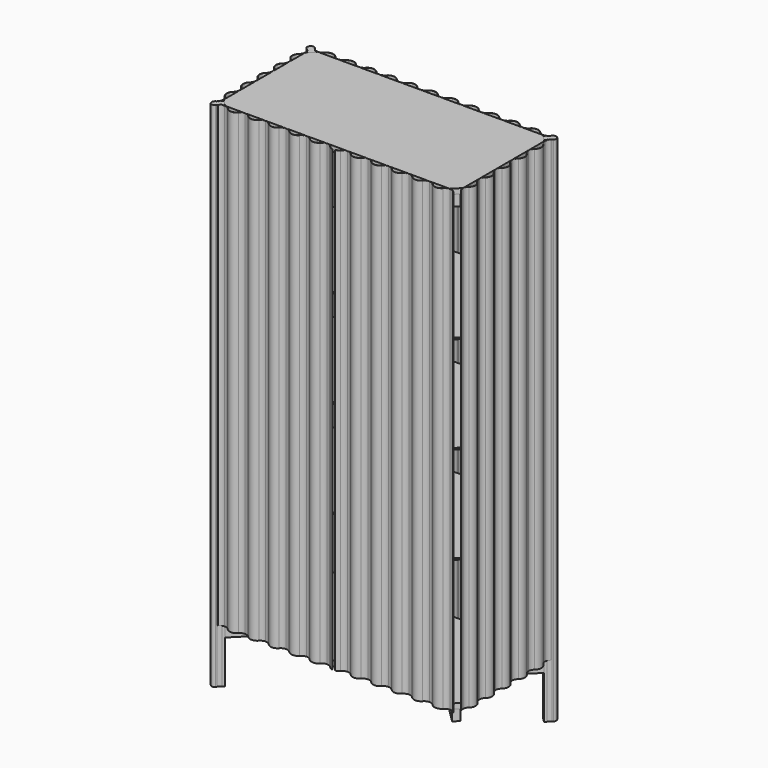
from build123d import *

# Parameters (mm, degrees)
F1_DEPTH       = 1700
F1_DEPTH_BACK  = 200
F2_DEPTH       = 1700
F4_DEPTH       = 19
F7_DEPTH       = 40
F8_DEPTH       = 40
F12_DEPTH      = 3
F12_DEPTH_BACK = 3
F15_R          = 2
F16_DEPTH      = 341.9145833847
F16_DEPTH_BACK = 642.3552756058


# Not quite as in the source:
# - a feature names something its author has since deleted; it is built from what else it names


with BuildPart() as f1:
    # F0 (on Top) → F1 (new body, two sides)
    with BuildSketch(Plane.XY) as f1_sk:
        with BuildLine():
            Line((-444.1128755262, -200.5565263401), (-451.3698203647, -207.8134711786))
            Line((-451.3698203647, -207.8134711786), (-454.0123704628, -210.4560212767))
            Line((-454.0123704628, -210.4560212767), (-455.0730306346, -209.3953611049))
            Line((-455.0730306346, -209.3953611049), (-458.3300735629, -212.6524040333))
            ThreePointArc((-458.3300735629, -212.6524040333), (-458.3300735629, -230.3300735629), (-440.6524040333, -230.3300735629))
            Line((-440.6524040333, -230.3300735629), (-437.3953611049, -227.0730306346))
            Line((-437.3953611049, -227.0730306346), (-438.4560212767, -226.0123704628))
            Line((-438.4560212767, -226.0123704628), (-435.8134706741, -223.3698198602))
            Line((-435.8134706741, -223.3698198602), (-428.5565263401, -216.1128755262))
            Line((-428.5565263401, -216.1128755262), (-427.4958661683, -217.1735356979))
            Line((-427.4958661683, -217.1735356979), (-421.2069675506, -210.8846370803))
            Line((-421.2069675506, -210.8846370803), (-438.8846370803, -193.2069675506))
            Line((-438.8846370803, -193.2069675506), (-445.1735356979, -199.4958661683))
            Line((-445.1735356979, -199.4958661683), (-444.1128755262, -200.5565263401))
        make_face()
    extrude(amount=F1_DEPTH)
    extrude(f1_sk.sketch, amount=-F1_DEPTH_BACK)


with BuildPart() as f1b:
    # F0 (on Top) → F1, piece 2 (new body, two sides)
    with BuildSketch(Plane.XY) as f1_2_sk:
        with BuildLine():
            Line((-428.5565263401, 216.1128755262), (-435.8134706741, 223.3698198602))
            Line((-435.8134706741, 223.3698198602), (-438.4560212767, 226.0123704628))
            Line((-438.4560212767, 226.0123704628), (-437.3953611049, 227.0730306346))
            Line((-437.3953611049, 227.0730306346), (-440.6524040333, 230.3300735629))
            ThreePointArc((-440.6524040333, 230.3300735629), (-458.3300735629, 230.3300735629), (-458.3300735629, 212.6524040333))
            Line((-458.3300735629, 212.6524040333), (-455.0730306346, 209.3953611049))
            Line((-455.0730306346, 209.3953611049), (-454.0123704628, 210.4560212767))
            Line((-454.0123704628, 210.4560212767), (-451.3698200275, 207.8134708414))
            Line((-451.3698200275, 207.8134708414), (-444.1128755262, 200.5565263401))
            Line((-444.1128755262, 200.5565263401), (-445.1735356979, 199.4958661683))
            Line((-445.1735356979, 199.4958661683), (-438.8846370803, 193.2069675506))
            Line((-438.8846370803, 193.2069675506), (-421.2069675506, 210.8846370803))
            Line((-421.2069675506, 210.8846370803), (-427.4958661683, 217.1735356979))
            Line((-427.4958661683, 217.1735356979), (-428.5565263401, 216.1128755262))
        make_face()
    extrude(amount=F1_DEPTH)
    extrude(f1_2_sk.sketch, amount=-F1_DEPTH_BACK)


with BuildPart() as f1c:
    # F0 (on Top) → F1, piece 3 (new body, two sides)
    with BuildSketch(Plane.XY) as f1_3_sk:
        with BuildLine():
            Line((438.4560212767, 226.0123704628), (435.8134711117, 223.3698202978))
            Line((435.8134711117, 223.3698202978), (428.5565263401, 216.1128755262))
            Line((428.5565263401, 216.1128755262), (427.4958661683, 217.1735356979))
            Line((427.4958661683, 217.1735356979), (421.2069675506, 210.8846370803))
            Line((421.2069675506, 210.8846370803), (438.8846370803, 193.2069675506))
            Line((438.8846370803, 193.2069675506), (445.1735356979, 199.4958661683))
            Line((445.1735356979, 199.4958661683), (444.1128755262, 200.5565263401))
            Line((444.1128755262, 200.5565263401), (451.3698203996, 207.8134712135))
            Line((451.3698203996, 207.8134712135), (454.0123704628, 210.4560212767))
            Line((454.0123704628, 210.4560212767), (455.0730306346, 209.3953611049))
            Line((455.0730306346, 209.3953611049), (458.3300735629, 212.6524040333))
            ThreePointArc((458.3300735629, 212.6524040333), (458.3300735629, 230.3300735629), (440.6524040333, 230.3300735629))
            Line((440.6524040333, 230.3300735629), (437.3953611049, 227.0730306346))
            Line((437.3953611049, 227.0730306346), (438.4560212767, 226.0123704628))
        make_face()
    extrude(amount=F1_DEPTH)
    extrude(f1_3_sk.sketch, amount=-F1_DEPTH_BACK)


with BuildPart() as f2:
    # F0 (on Top) → F2 (new body)
    with BuildSketch(Plane.XY):
        with BuildLine():
            ThreePointArc((418, -216.6912387981), (428.1481401623, -218.8925783259), (436.4720557108, -225.1008852138))
            Line((436.4720557108, -225.1008852138), (437, -224.6412387981))
            ThreePointArc((437, -224.6412387981), (428.4381811155, -218.2554941513), (418, -215.9912387981))
            ThreePointArc((418, -215.9912387981), (407.5618188845, -218.2554941513), (399, -224.6412387981))
            ThreePointArc((399, -224.6412387981), (380, -233.2912387981), (361, -224.6412387981))
            ThreePointArc((361, -224.6412387981), (352.4381811155, -218.2554941513), (342, -215.9912387981))
            ThreePointArc((342, -215.9912387981), (331.5618188845, -218.2554941513), (323, -224.6412387981))
            ThreePointArc((323, -224.6412387981), (304, -233.2912387981), (285, -224.6412387981))
            ThreePointArc((285, -224.6412387981), (276.4381811155, -218.2554941513), (266, -215.9912387981))
            ThreePointArc((266, -215.9912387981), (255.5618188845, -218.2554941513), (247, -224.6412387981))
            ThreePointArc((247, -224.6412387981), (228, -233.2912387981), (209, -224.6412387981))
            ThreePointArc((209, -224.6412387981), (200.4381811155, -218.2554941513), (190, -215.9912387981))
            ThreePointArc((190, -215.9912387981), (179.5618188845, -218.2554941513), (171, -224.6412387981))
            ThreePointArc((171, -224.6412387981), (152, -233.2912387981), (133, -224.6412387981))
            ThreePointArc((133, -224.6412387981), (124.4381811155, -218.2554941513), (114, -215.9912387981))
            ThreePointArc((114, -215.9912387981), (103.5618188845, -218.2554941513), (95, -224.6412387981))
            ThreePointArc((95, -224.6412387981), (76, -233.2912387981), (57, -224.6412387981))
            ThreePointArc((57, -224.6412387981), (48.4381811155, -218.2554941513), (38, -215.9912387981))
            ThreePointArc((38, -215.9912387981), (27.5618188845, -218.2554941513), (19, -224.6412387981))
            ThreePointArc((19, -224.6412387981), (12.6728388126, -229.8716152469), (5, -232.7900653567))
            Line((5, -232.7900653567), (5, -233.5038784277))
            ThreePointArc((5, -233.5038784277), (12.963702654, -230.5121466747), (19.5279442892, -225.1008852138))
            ThreePointArc((19.5279442892, -225.1008852138), (27.8518598377, -218.8925783259), (38, -216.6912387981))
            ThreePointArc((38, -216.6912387981), (48.1481401623, -218.8925783259), (56.4720557108, -225.1008852138))
            ThreePointArc((56.4720557108, -225.1008852138), (76, -233.9912387981), (95.5279442892, -225.1008852138))
            ThreePointArc((95.5279442892, -225.1008852138), (103.8518598377, -218.8925783259), (114, -216.6912387981))
            ThreePointArc((114, -216.6912387981), (124.1481401623, -218.8925783259), (132.4720557108, -225.1008852138))
            ThreePointArc((132.4720557108, -225.1008852138), (152, -233.9912387981), (171.5279442892, -225.1008852138))
            ThreePointArc((171.5279442892, -225.1008852138), (179.8518598377, -218.8925783259), (190, -216.6912387981))
            ThreePointArc((190, -216.6912387981), (200.1481401623, -218.8925783259), (208.4720557108, -225.1008852138))
            ThreePointArc((208.4720557108, -225.1008852138), (228, -233.9912387981), (247.5279442892, -225.1008852138))
            ThreePointArc((247.5279442892, -225.1008852138), (255.8518598377, -218.8925783259), (266, -216.6912387981))
            ThreePointArc((266, -216.6912387981), (276.1481401623, -218.8925783259), (284.4720557108, -225.1008852138))
            ThreePointArc((284.4720557108, -225.1008852138), (304, -233.9912387981), (323.5279442892, -225.1008852138))
            ThreePointArc((323.5279442892, -225.1008852138), (331.8518598377, -218.8925783259), (342, -216.6912387981))
            ThreePointArc((342, -216.6912387981), (352.1481401623, -218.8925783259), (360.4720557108, -225.1008852138))
            ThreePointArc((360.4720557108, -225.1008852138), (380, -233.9912387981), (399.5279442892, -225.1008852138))
            ThreePointArc((399.5279442892, -225.1008852138), (407.8518598377, -218.8925783259), (418, -216.6912387981))
        make_face()
    extrude(amount=F2_DEPTH)


with BuildPart() as f2b:
    # F0 (on Top) → F2, piece 2 (new body)
    with BuildSketch(Plane.XY):
        with BuildLine():
            ThreePointArc((-418, -215.9912387981), (-427.6405808428, -217.9088695363), (-435.8134706741, -223.3698198602))
            ThreePointArc((-435.8134706741, -223.3698198602), (-436.4177097462, -223.9952876551), (-437, -224.6412387981))
            Line((-437, -224.6412387981), (-436.4720557108, -225.1008852138))
            ThreePointArc((-436.4720557108, -225.1008852138), (-428.1481401623, -218.8925783259), (-418, -216.6912387981))
            ThreePointArc((-418, -216.6912387981), (-407.8518598377, -218.8925783259), (-399.5279442892, -225.1008852138))
            ThreePointArc((-399.5279442892, -225.1008852138), (-380, -233.9912387981), (-360.4720557108, -225.1008852138))
            ThreePointArc((-360.4720557108, -225.1008852138), (-352.1481401623, -218.8925783259), (-342, -216.6912387981))
            ThreePointArc((-342, -216.6912387981), (-331.8518598377, -218.8925783259), (-323.5279442892, -225.1008852138))
            ThreePointArc((-323.5279442892, -225.1008852138), (-304, -233.9912387981), (-284.4720557108, -225.1008852138))
            ThreePointArc((-284.4720557108, -225.1008852138), (-276.1481401623, -218.8925783259), (-266, -216.6912387981))
            ThreePointArc((-266, -216.6912387981), (-255.8518598377, -218.8925783259), (-247.5279442892, -225.1008852138))
            ThreePointArc((-247.5279442892, -225.1008852138), (-228, -233.9912387981), (-208.4720557108, -225.1008852138))
            ThreePointArc((-208.4720557108, -225.1008852138), (-200.1481401623, -218.8925783259), (-190, -216.6912387981))
            ThreePointArc((-190, -216.6912387981), (-179.8518598377, -218.8925783259), (-171.5279442892, -225.1008852138))
            ThreePointArc((-171.5279442892, -225.1008852138), (-152, -233.9912387981), (-132.4720557108, -225.1008852138))
            ThreePointArc((-132.4720557108, -225.1008852138), (-124.1481401623, -218.8925783259), (-114, -216.6912387981))
            ThreePointArc((-114, -216.6912387981), (-103.8518598377, -218.8925783259), (-95.5279442892, -225.1008852138))
            ThreePointArc((-95.5279442892, -225.1008852138), (-76, -233.9912387981), (-56.4720557108, -225.1008852138))
            ThreePointArc((-56.4720557108, -225.1008852138), (-48.1481401623, -218.8925783259), (-38, -216.6912387981))
            ThreePointArc((-38, -216.6912387981), (-27.8518598377, -218.8925783259), (-19.5279442892, -225.1008852138))
            ThreePointArc((-19.5279442892, -225.1008852138), (-12.963702654, -230.5121466747), (-5, -233.5038784277))
            Line((-5, -233.5038784277), (-5, -232.7900653567))
            ThreePointArc((-5, -232.7900653567), (-12.6728388126, -229.8716152469), (-19, -224.6412387981))
            ThreePointArc((-19, -224.6412387981), (-27.5618188845, -218.2554941513), (-38, -215.9912387981))
            ThreePointArc((-38, -215.9912387981), (-48.4381811155, -218.2554941513), (-57, -224.6412387981))
            ThreePointArc((-57, -224.6412387981), (-76, -233.2912387981), (-95, -224.6412387981))
            ThreePointArc((-95, -224.6412387981), (-103.5618188845, -218.2554941513), (-114, -215.9912387981))
            ThreePointArc((-114, -215.9912387981), (-124.4381811155, -218.2554941513), (-133, -224.6412387981))
            ThreePointArc((-133, -224.6412387981), (-152, -233.2912387981), (-171, -224.6412387981))
            ThreePointArc((-171, -224.6412387981), (-179.5618188845, -218.2554941513), (-190, -215.9912387981))
            ThreePointArc((-190, -215.9912387981), (-200.4381811155, -218.2554941513), (-209, -224.6412387981))
            ThreePointArc((-209, -224.6412387981), (-228, -233.2912387981), (-247, -224.6412387981))
            ThreePointArc((-247, -224.6412387981), (-255.5618188845, -218.2554941513), (-266, -215.9912387981))
            ThreePointArc((-266, -215.9912387981), (-276.4381811155, -218.2554941513), (-285, -224.6412387981))
            ThreePointArc((-285, -224.6412387981), (-304, -233.2912387981), (-323, -224.6412387981))
            ThreePointArc((-323, -224.6412387981), (-331.5618188845, -218.2554941513), (-342, -215.9912387981))
            ThreePointArc((-342, -215.9912387981), (-352.4381811155, -218.2554941513), (-361, -224.6412387981))
            ThreePointArc((-361, -224.6412387981), (-380, -233.2912387981), (-399, -224.6412387981))
            ThreePointArc((-399, -224.6412387981), (-407.5618188845, -218.2554941513), (-418, -215.9912387981))
        make_face()
    extrude(amount=F2_DEPTH)


with BuildPart() as f2c:
    # F0 (on Top) → F2, piece 3 (new body)
    with BuildSketch(Plane.XY):
        with BuildLine():
            ThreePointArc((-443.9912387981, 190), (-445.9088695815, 199.6405809521), (-451.3698200275, 207.8134708414))
            ThreePointArc((-451.3698200275, 207.8134708414), (-451.9952877416, 208.417709827), (-452.6412387981, 209))
            Line((-452.6412387981, 209), (-453.1008852138, 208.4720557108))
            ThreePointArc((-453.1008852138, 208.4720557108), (-446.8925783259, 200.1481401623), (-444.6912387981, 190))
            ThreePointArc((-444.6912387981, 190), (-446.8925783259, 179.8518598377), (-453.1008852138, 171.5279442892))
            ThreePointArc((-453.1008852138, 171.5279442892), (-461.9912387981, 152), (-453.1008852138, 132.4720557108))
            ThreePointArc((-453.1008852138, 132.4720557108), (-446.8925783259, 124.1481401623), (-444.6912387981, 114))
            ThreePointArc((-444.6912387981, 114), (-446.8925783259, 103.8518598377), (-453.1008852138, 95.5279442892))
            ThreePointArc((-453.1008852138, 95.5279442892), (-461.9912387981, 76), (-453.1008852138, 56.4720557108))
            ThreePointArc((-453.1008852138, 56.4720557108), (-446.8925783259, 48.1481401623), (-444.6912387981, 38))
            ThreePointArc((-444.6912387981, 38), (-446.8925783259, 27.8518598377), (-453.1008852138, 19.5279442892))
            ThreePointArc((-453.1008852138, 19.5279442892), (-461.9912387981, 0), (-453.1008852138, -19.5279442892))
            ThreePointArc((-453.1008852138, -19.5279442892), (-446.8925783259, -27.8518598377), (-444.6912387981, -38))
            ThreePointArc((-444.6912387981, -38), (-446.8925783259, -48.1481401623), (-453.1008852138, -56.4720557108))
            ThreePointArc((-453.1008852138, -56.4720557108), (-461.9912387981, -76), (-453.1008852138, -95.5279442892))
            ThreePointArc((-453.1008852138, -95.5279442892), (-446.8925783259, -103.8518598377), (-444.6912387981, -114))
            ThreePointArc((-444.6912387981, -114), (-446.8925783259, -124.1481401623), (-453.1008852138, -132.4720557108))
            ThreePointArc((-453.1008852138, -132.4720557108), (-461.9912387981, -152), (-453.1008852138, -171.5279442892))
            ThreePointArc((-453.1008852138, -171.5279442892), (-446.8925783259, -179.8518598377), (-444.6912387981, -190))
            ThreePointArc((-444.6912387981, -190), (-446.8925783259, -200.1481401623), (-453.1008852138, -208.4720557108))
            Line((-453.1008852138, -208.4720557108), (-452.6412387981, -209))
            ThreePointArc((-452.6412387981, -209), (-451.9952879159, -208.4177099896), (-451.3698203647, -207.8134711786))
            ThreePointArc((-451.3698203647, -207.8134711786), (-445.9088696728, -199.6405811724), (-443.9912387981, -190))
            ThreePointArc((-443.9912387981, -190), (-446.2554941513, -179.5618188845), (-452.6412387981, -171))
            ThreePointArc((-452.6412387981, -171), (-461.2912387981, -152), (-452.6412387981, -133))
            ThreePointArc((-452.6412387981, -133), (-446.2554941513, -124.4381811155), (-443.9912387981, -114))
            ThreePointArc((-443.9912387981, -114), (-446.2554941513, -103.5618188845), (-452.6412387981, -95))
            ThreePointArc((-452.6412387981, -95), (-461.2912387981, -76), (-452.6412387981, -57))
            ThreePointArc((-452.6412387981, -57), (-446.2554941513, -48.4381811155), (-443.9912387981, -38))
            ThreePointArc((-443.9912387981, -38), (-446.2554941513, -27.5618188845), (-452.6412387981, -19))
            ThreePointArc((-452.6412387981, -19), (-461.2912387981, 0), (-452.6412387981, 19))
            ThreePointArc((-452.6412387981, 19), (-446.2554941513, 27.5618188845), (-443.9912387981, 38))
            ThreePointArc((-443.9912387981, 38), (-446.2554941513, 48.4381811155), (-452.6412387981, 57))
            ThreePointArc((-452.6412387981, 57), (-461.2912387981, 76), (-452.6412387981, 95))
            ThreePointArc((-452.6412387981, 95), (-446.2554941513, 103.5618188845), (-443.9912387981, 114))
            ThreePointArc((-443.9912387981, 114), (-446.2554941513, 124.4381811155), (-452.6412387981, 133))
            ThreePointArc((-452.6412387981, 133), (-461.2912387981, 152), (-452.6412387981, 171))
            ThreePointArc((-452.6412387981, 171), (-446.2554941513, 179.5618188845), (-443.9912387981, 190))
        make_face()
    extrude(amount=F2_DEPTH)


with BuildPart() as f2d:
    # F0 (on Top) → F2, piece 4 (new body)
    with BuildSketch(Plane.XY):
        with BuildLine():
            ThreePointArc((0, 233.2912387981), (10.4381811155, 231.0269834449), (19, 224.6412387981))
            ThreePointArc((19, 224.6412387981), (27.5618188845, 218.2554941513), (38, 215.9912387981))
            ThreePointArc((38, 215.9912387981), (48.4381811155, 218.2554941513), (57, 224.6412387981))
            ThreePointArc((57, 224.6412387981), (76, 233.2912387981), (95, 224.6412387981))
            ThreePointArc((95, 224.6412387981), (103.5618188845, 218.2554941513), (114, 215.9912387981))
            ThreePointArc((114, 215.9912387981), (124.4381811155, 218.2554941513), (133, 224.6412387981))
            ThreePointArc((133, 224.6412387981), (152, 233.2912387981), (171, 224.6412387981))
            ThreePointArc((171, 224.6412387981), (179.5618188845, 218.2554941513), (190, 215.9912387981))
            ThreePointArc((190, 215.9912387981), (200.4381811155, 218.2554941513), (209, 224.6412387981))
            ThreePointArc((209, 224.6412387981), (228, 233.2912387981), (247, 224.6412387981))
            ThreePointArc((247, 224.6412387981), (255.5618188845, 218.2554941513), (266, 215.9912387981))
            ThreePointArc((266, 215.9912387981), (276.4381811155, 218.2554941513), (285, 224.6412387981))
            ThreePointArc((285, 224.6412387981), (304, 233.2912387981), (323, 224.6412387981))
            ThreePointArc((323, 224.6412387981), (331.5618188845, 218.2554941513), (342, 215.9912387981))
            ThreePointArc((342, 215.9912387981), (352.4381811155, 218.2554941513), (361, 224.6412387981))
            ThreePointArc((361, 224.6412387981), (380, 233.2912387981), (399, 224.6412387981))
            ThreePointArc((399, 224.6412387981), (407.5618188845, 218.2554941513), (418, 215.9912387981))
            ThreePointArc((418, 215.9912387981), (427.6405811287, 217.9088696547), (435.8134711117, 223.3698202978))
            ThreePointArc((435.8134711117, 223.3698202978), (436.4177099574, 223.9952878813), (437, 224.6412387981))
            Line((437, 224.6412387981), (436.4720557108, 225.1008852138))
            ThreePointArc((436.4720557108, 225.1008852138), (428.1481401623, 218.8925783259), (418, 216.6912387981))
            ThreePointArc((418, 216.6912387981), (407.8518598377, 218.8925783259), (399.5279442892, 225.1008852138))
            ThreePointArc((399.5279442892, 225.1008852138), (380, 233.9912387981), (360.4720557108, 225.1008852138))
            ThreePointArc((360.4720557108, 225.1008852138), (352.1481401623, 218.8925783259), (342, 216.6912387981))
            ThreePointArc((342, 216.6912387981), (331.8518598377, 218.8925783259), (323.5279442892, 225.1008852138))
            ThreePointArc((323.5279442892, 225.1008852138), (304, 233.9912387981), (284.4720557108, 225.1008852138))
            ThreePointArc((284.4720557108, 225.1008852138), (276.1481401623, 218.8925783259), (266, 216.6912387981))
            ThreePointArc((266, 216.6912387981), (255.8518598377, 218.8925783259), (247.5279442892, 225.1008852138))
            ThreePointArc((247.5279442892, 225.1008852138), (228, 233.9912387981), (208.4720557108, 225.1008852138))
            ThreePointArc((208.4720557108, 225.1008852138), (200.1481401623, 218.8925783259), (190, 216.6912387981))
            ThreePointArc((190, 216.6912387981), (179.8518598377, 218.8925783259), (171.5279442892, 225.1008852138))
            ThreePointArc((171.5279442892, 225.1008852138), (152, 233.9912387981), (132.4720557108, 225.1008852138))
            ThreePointArc((132.4720557108, 225.1008852138), (124.1481401623, 218.8925783259), (114, 216.6912387981))
            ThreePointArc((114, 216.6912387981), (103.8518598377, 218.8925783259), (95.5279442892, 225.1008852138))
            ThreePointArc((95.5279442892, 225.1008852138), (76, 233.9912387981), (56.4720557108, 225.1008852138))
            ThreePointArc((56.4720557108, 225.1008852138), (48.1481401623, 218.8925783259), (38, 216.6912387981))
            ThreePointArc((38, 216.6912387981), (27.8518598377, 218.8925783259), (19.5279442892, 225.1008852138))
            ThreePointArc((19.5279442892, 225.1008852138), (10.7282220687, 231.6640676194), (0, 233.9912387981))
            ThreePointArc((0, 233.9912387981), (-10.7282220687, 231.6640676194), (-19.5279442892, 225.1008852138))
            ThreePointArc((-19.5279442892, 225.1008852138), (-27.8518598377, 218.8925783259), (-38, 216.6912387981))
            ThreePointArc((-38, 216.6912387981), (-48.1481401623, 218.8925783259), (-56.4720557108, 225.1008852138))
            ThreePointArc((-56.4720557108, 225.1008852138), (-76, 233.9912387981), (-95.5279442892, 225.1008852138))
            ThreePointArc((-95.5279442892, 225.1008852138), (-103.8518598377, 218.8925783259), (-114, 216.6912387981))
            ThreePointArc((-114, 216.6912387981), (-124.1481401623, 218.8925783259), (-132.4720557108, 225.1008852138))
            ThreePointArc((-132.4720557108, 225.1008852138), (-152, 233.9912387981), (-171.5279442892, 225.1008852138))
            ThreePointArc((-171.5279442892, 225.1008852138), (-179.8518598377, 218.8925783259), (-190, 216.6912387981))
            ThreePointArc((-190, 216.6912387981), (-200.1481401623, 218.8925783259), (-208.4720557108, 225.1008852138))
            ThreePointArc((-208.4720557108, 225.1008852138), (-228, 233.9912387981), (-247.5279442892, 225.1008852138))
            ThreePointArc((-247.5279442892, 225.1008852138), (-255.8518598377, 218.8925783259), (-266, 216.6912387981))
            ThreePointArc((-266, 216.6912387981), (-276.1481401623, 218.8925783259), (-284.4720557108, 225.1008852138))
            ThreePointArc((-284.4720557108, 225.1008852138), (-304, 233.9912387981), (-323.5279442892, 225.1008852138))
            ThreePointArc((-323.5279442892, 225.1008852138), (-331.8518598377, 218.8925783259), (-342, 216.6912387981))
            ThreePointArc((-342, 216.6912387981), (-352.1481401623, 218.8925783259), (-360.4720557108, 225.1008852138))
            ThreePointArc((-360.4720557108, 225.1008852138), (-380, 233.9912387981), (-399.5279442892, 225.1008852138))
            ThreePointArc((-399.5279442892, 225.1008852138), (-407.8518598377, 218.8925783259), (-418, 216.6912387981))
            ThreePointArc((-418, 216.6912387981), (-428.1481401623, 218.8925783259), (-436.4720557108, 225.1008852138))
            Line((-436.4720557108, 225.1008852138), (-437, 224.6412387981))
            ThreePointArc((-437, 224.6412387981), (-436.4177097462, 223.9952876551), (-435.8134706741, 223.3698198602))
            ThreePointArc((-435.8134706741, 223.3698198602), (-427.6405808428, 217.9088695363), (-418, 215.9912387981))
            ThreePointArc((-418, 215.9912387981), (-407.5618188845, 218.2554941513), (-399, 224.6412387981))
            ThreePointArc((-399, 224.6412387981), (-380, 233.2912387981), (-361, 224.6412387981))
            ThreePointArc((-361, 224.6412387981), (-352.4381811155, 218.2554941513), (-342, 215.9912387981))
            ThreePointArc((-342, 215.9912387981), (-331.5618188845, 218.2554941513), (-323, 224.6412387981))
            ThreePointArc((-323, 224.6412387981), (-304, 233.2912387981), (-285, 224.6412387981))
            ThreePointArc((-285, 224.6412387981), (-276.4381811155, 218.2554941513), (-266, 215.9912387981))
            ThreePointArc((-266, 215.9912387981), (-255.5618188845, 218.2554941513), (-247, 224.6412387981))
            ThreePointArc((-247, 224.6412387981), (-228, 233.2912387981), (-209, 224.6412387981))
            ThreePointArc((-209, 224.6412387981), (-200.4381811155, 218.2554941513), (-190, 215.9912387981))
            ThreePointArc((-190, 215.9912387981), (-179.5618188845, 218.2554941513), (-171, 224.6412387981))
            ThreePointArc((-171, 224.6412387981), (-152, 233.2912387981), (-133, 224.6412387981))
            ThreePointArc((-133, 224.6412387981), (-124.4381811155, 218.2554941513), (-114, 215.9912387981))
            ThreePointArc((-114, 215.9912387981), (-103.5618188845, 218.2554941513), (-95, 224.6412387981))
            ThreePointArc((-95, 224.6412387981), (-76, 233.2912387981), (-57, 224.6412387981))
            ThreePointArc((-57, 224.6412387981), (-48.4381811155, 218.2554941513), (-38, 215.9912387981))
            ThreePointArc((-38, 215.9912387981), (-27.5618188845, 218.2554941513), (-19, 224.6412387981))
            ThreePointArc((-19, 224.6412387981), (-10.4381811155, 231.0269834449), (0, 233.2912387981))
        make_face()
    extrude(amount=F2_DEPTH)


with BuildPart() as f2e:
    # F0 (on Top) → F2, piece 5 (new body)
    with BuildSketch(Plane.XY):
        with BuildLine():
            ThreePointArc((452.6412387981, 209), (451.9952879339, 208.4177100065), (451.3698203996, 207.8134712135))
            ThreePointArc((451.3698203996, 207.8134712135), (445.9088696822, 199.6405811952), (443.9912387981, 190))
            ThreePointArc((443.9912387981, 190), (446.2554941513, 179.5618188845), (452.6412387981, 171))
            ThreePointArc((452.6412387981, 171), (461.2912387981, 152), (452.6412387981, 133))
            ThreePointArc((452.6412387981, 133), (446.2554941513, 124.4381811155), (443.9912387981, 114))
            ThreePointArc((443.9912387981, 114), (446.2554941513, 103.5618188845), (452.6412387981, 95))
            ThreePointArc((452.6412387981, 95), (461.2912387981, 76), (452.6412387981, 57))
            ThreePointArc((452.6412387981, 57), (446.2554941513, 48.4381811155), (443.9912387981, 38))
            ThreePointArc((443.9912387981, 38), (446.2554941513, 27.5618188845), (452.6412387981, 19))
            ThreePointArc((452.6412387981, 19), (461.2912387981, 0), (452.6412387981, -19))
            ThreePointArc((452.6412387981, -19), (446.2554941513, -27.5618188845), (443.9912387981, -38))
            ThreePointArc((443.9912387981, -38), (446.2554941513, -48.4381811155), (452.6412387981, -57))
            ThreePointArc((452.6412387981, -57), (461.2912387981, -76), (452.6412387981, -95))
            ThreePointArc((452.6412387981, -95), (446.2554941513, -103.5618188845), (443.9912387981, -114))
            ThreePointArc((443.9912387981, -114), (446.2554941513, -124.4381811155), (452.6412387981, -133))
            ThreePointArc((452.6412387981, -133), (461.2912387981, -152), (452.6412387981, -171))
            ThreePointArc((452.6412387981, -171), (446.2554941513, -179.5618188845), (443.9912387981, -190))
            ThreePointArc((443.9912387981, -190), (445.9088695363, -199.6405808428), (451.3698198602, -207.8134706741))
            ThreePointArc((451.3698198602, -207.8134706741), (451.9952876551, -208.4177097462), (452.6412387981, -209))
            Line((452.6412387981, -209), (453.1008852138, -208.4720557108))
            ThreePointArc((453.1008852138, -208.4720557108), (446.8925783259, -200.1481401623), (444.6912387981, -190))
            ThreePointArc((444.6912387981, -190), (446.8925783259, -179.8518598377), (453.1008852138, -171.5279442892))
            ThreePointArc((453.1008852138, -171.5279442892), (461.9912387981, -152), (453.1008852138, -132.4720557108))
            ThreePointArc((453.1008852138, -132.4720557108), (446.8925783259, -124.1481401623), (444.6912387981, -114))
            ThreePointArc((444.6912387981, -114), (446.8925783259, -103.8518598377), (453.1008852138, -95.5279442892))
            ThreePointArc((453.1008852138, -95.5279442892), (461.9912387981, -76), (453.1008852138, -56.4720557108))
            ThreePointArc((453.1008852138, -56.4720557108), (446.8925783259, -48.1481401623), (444.6912387981, -38))
            ThreePointArc((444.6912387981, -38), (446.8925783259, -27.8518598377), (453.1008852138, -19.5279442892))
            ThreePointArc((453.1008852138, -19.5279442892), (461.9912387981, 0), (453.1008852138, 19.5279442892))
            ThreePointArc((453.1008852138, 19.5279442892), (446.8925783259, 27.8518598377), (444.6912387981, 38))
            ThreePointArc((444.6912387981, 38), (446.8925783259, 48.1481401623), (453.1008852138, 56.4720557108))
            ThreePointArc((453.1008852138, 56.4720557108), (461.9912387981, 76), (453.1008852138, 95.5279442892))
            ThreePointArc((453.1008852138, 95.5279442892), (446.8925783259, 103.8518598377), (444.6912387981, 114))
            ThreePointArc((444.6912387981, 114), (446.8925783259, 124.1481401623), (453.1008852138, 132.4720557108))
            ThreePointArc((453.1008852138, 132.4720557108), (461.9912387981, 152), (453.1008852138, 171.5279442892))
            ThreePointArc((453.1008852138, 171.5279442892), (446.8925783259, 179.8518598377), (444.6912387981, 190))
            ThreePointArc((444.6912387981, 190), (446.8925783259, 200.1481401623), (453.1008852138, 208.4720557108))
            Line((453.1008852138, 208.4720557108), (452.6412387981, 209))
        make_face()
    extrude(amount=F2_DEPTH)


with BuildPart() as f4:
    # F3 (on face) → F4 (new body)
    with BuildSketch(Plane(origin=(0, 0, 0), x_dir=(1, 0, 0), z_dir=(0, 0, -1))):
        Polygon((-416.0226432972, 216.0689613337), (-443.9912387981, 188.1003658328), (-443.9912387981, -188.1003658328), (-416.1003658328, -215.9912387981), (416.1003658328, -215.9912387981), (443.9912387981, -188.1003658328), (443.9912387981, 188.1003658328), (416.3088630935, 215.7827415374), align=None)
    extrude(amount=-F4_DEPTH)


with BuildPart() as f5_1:
    # F5: copy of F4
    add(f4.part.moved(Location((0, 0, 1681))))


with BuildPart() as f7:
    # F6 (on face) → F7 (new body)
    with BuildSketch(Plane(origin=(0, 0, 0), x_dir=(1, 0, 0), z_dir=(0, 0, -1))):
        Polygon((-421.2069675506, -210.8846370803), (-228, -17.6776695297), (-245.6776695297, 0), (-438.8846370803, -193.2069675506), align=None)
    extrude(amount=F7_DEPTH)


with BuildPart() as f7b:
    # F6 (on face) → F7, piece 2 (new body)
    with BuildSketch(Plane(origin=(0, 0, 0), x_dir=(1, 0, 0), z_dir=(0, 0, -1))):
        Polygon((228, -17.6776695297), (421.2069675506, -210.8846370803), (438.8846370803, -193.2069675506), (245.6776695297, 0), align=None)
    extrude(amount=F7_DEPTH)


with BuildPart() as f8:
    # F6 (on face) → F8 (new body, through all)
    with BuildSketch(Plane(origin=(0, 0, 0), x_dir=(1, 0, 0), z_dir=(0, 0, -1))):
        Polygon((-228, -17.6776695297), (-210.3223304703, 0), (-421.2069675506, 210.8846370803), (-438.8846370803, 193.2069675506), (-245.6776695297, 0), align=None)
    extrude(amount=F8_DEPTH)


with BuildPart() as f8b:
    # F6 (on face) → F8, piece 2 (new body, through all)
    with BuildSketch(Plane(origin=(0, 0, 0), x_dir=(1, 0, 0), z_dir=(0, 0, -1))):
        Polygon((438.8846370803, 193.2069675506), (421.2069675506, 210.8846370803), (210.3223304703, 0), (228, -17.6776695297), (245.6776695297, 0), align=None)
    extrude(amount=F8_DEPTH)


with BuildPart() as f9_1:
    # F9: copy of F7b
    add(f7b.part.moved(Location((0, 0, 1681))))


with BuildPart() as f9_2:
    # F9: copy of F8b
    add(f8b.part.moved(Location((0, 0, 1681))))


with BuildPart() as f9_3:
    # F9: copy of F7
    add(f7.part.moved(Location((0, 0, 1681))))


with BuildPart() as f9_4:
    # F9: copy of F8
    add(f8.part.moved(Location((0, 0, 1681))))


with BuildPart() as f12:
    # F11 (on mid) → F12 (new body, two sides)
    with BuildSketch(Plane.XY.offset(850)) as f12_sk:
        Polygon((419.7927539883, -212.2988506427), (443.9912387981, -188.1003658328), (443.9912387981, 188.1003658328), (416.1003658328, 215.9912387981), (-416.1003658328, 215.9912387981), (-443.9912387981, 188.1003658328), (-443.9912387981, -188.1003658328), align=None)
    extrude(amount=F12_DEPTH)
    extrude(f12_sk.sketch, amount=-F12_DEPTH_BACK)


with BuildPart() as f13_1:
    # F13: copy of F12
    add(f12.part.moved(Location((0, 0, 360))))


with BuildPart() as f14_1:
    # F14: copy of F12
    add(f12.part.moved(Location((0, 0, -360))))


with BuildPart() as f16_tool:
    # F15 (on face) → F16 (new body, two sides)
    with BuildSketch(Plane(origin=(-106.2218254069, -106.2218254069, 0), x_dir=(-0.7071067812, 0.7071067812, 0), z_dir=(0.7071067812, 0.7071067812, 0))) as f16_sk:
        with Locations((461.8501056831, 1600)):
            Circle(F15_R)
        with Locations((461.8501056831, 100)):
            Circle(F15_R)
    extrude(amount=-F16_DEPTH)
    extrude(f16_sk.sketch, amount=F16_DEPTH_BACK)


with BuildPart() as f1b_1:
    add(f1b.part)

    # F16: cut by f16_tool
    add(f16_tool.part, mode=Mode.SUBTRACT)


with BuildPart() as f2c_1:
    add(f2c.part)

    # F16: cut by f16_tool
    add(f16_tool.part, mode=Mode.SUBTRACT)


with BuildPart() as f2d_1:
    add(f2d.part)

    # F16: cut by f16_tool
    add(f16_tool.part, mode=Mode.SUBTRACT)


solid = Compound([f1.part, f1c.part, f2.part, f2b.part, f2e.part, f4.part, f5_1.part, f7.part, f7b.part, f8.part, f8b.part, f9_1.part, f9_2.part, f9_3.part, f9_4.part, f12.part, f13_1.part, f14_1.part, f1b_1.part, f2c_1.part, f2d_1.part])
